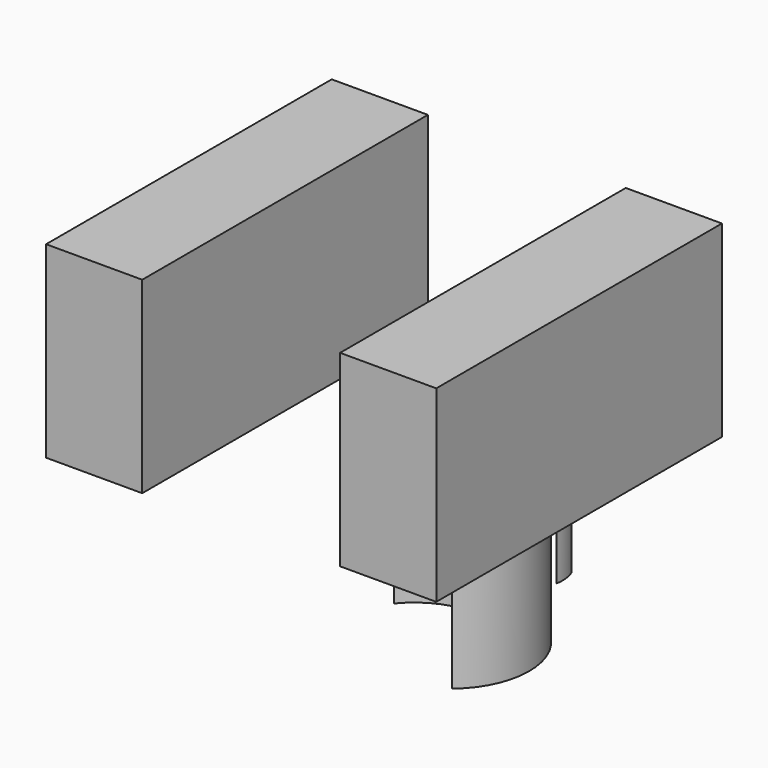
from build123d import *

# Parameters (mm, degrees)
F3_DEPTH      = 482.75577
F1_E0_RIGHT_W = 535.3775024414
F1_E0_RIGHT_H = 1017.07278
F4_DEPTH      = 273.88198
F1_E0_LEFT_W  = 535.3775024414
F1_E0_LEFT_H  = 1017.07278


with BuildPart() as f3:
    # F2 (on Top) → F3 (new body)
    with BuildSketch(Plane.XY):
        with BuildLine():
            ThreePointArc((189.9649500847, -357.6309978962), (477.4693061455, -315.2043475455), (547.0770597458, -597.3630547523))
            ThreePointArc((547.0770597458, -597.3630547523), (528.9406165931, -238.5311295286), (189.9649500847, -357.6309978962))
        make_face()
    extrude(amount=-F3_DEPTH)

    # F1_E0_right (on explicit) → F4 (join)
    with BuildSketch(Plane(origin=(837.4749422073, 0, 0), x_dir=(0, 0, 1), z_dir=(1, 0, 0))):
        with Locations((267.6887512207, 508.53639)):
            Rectangle(F1_E0_RIGHT_W, F1_E0_RIGHT_H)
    extrude(amount=-F4_DEPTH)


with BuildPart() as f3b:
    # F2 (on Top) → F3, piece 2 (new body)
    with BuildSketch(Plane.XY):
        with BuildLine():
            ThreePointArc((405.3064584732, 5.1124375314), (404.4428515066, -26.3399147003), (411.900691804, -56.9074938651))
            ThreePointArc((411.900691804, -56.9074938651), (412.8912838015, -25.4416400235), (405.3064584732, 5.1124375314))
        make_face()
    extrude(amount=-F3_DEPTH)


with BuildPart() as f4:
    # F1_E0_left (on explicit) → F4, piece 2 (new body)
    with BuildSketch(Plane(origin=(0, 0, 0), x_dir=(0, 0, 1), z_dir=(1, 0, 0))):
        with Locations((267.6887512207, 508.53639)):
            Rectangle(F1_E0_LEFT_W, F1_E0_LEFT_H)
    extrude(amount=-F4_DEPTH)


solid = Compound([f3.part, f3b.part, f4.part])
